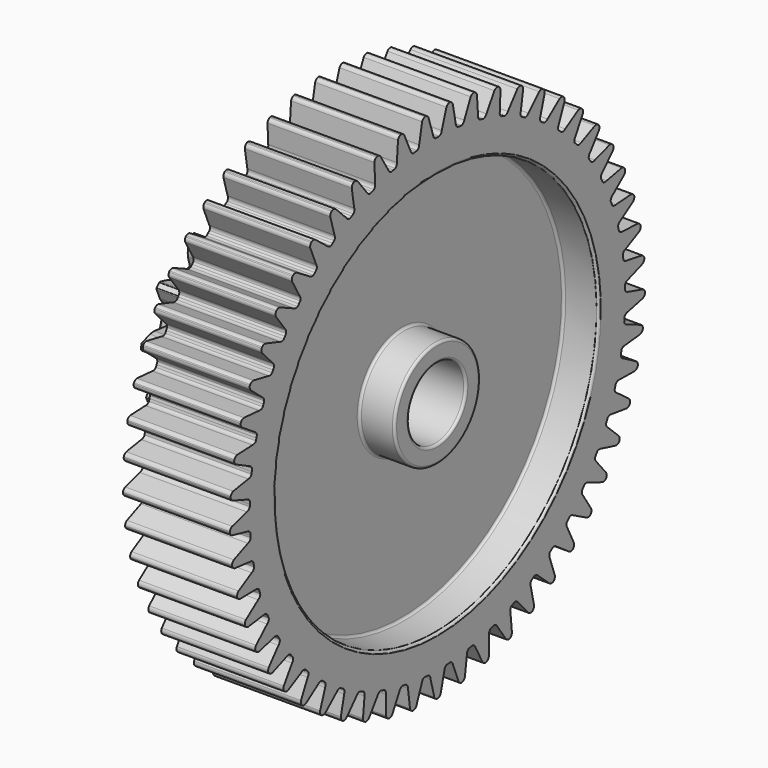
from build123d import *

# Parameters (mm, degrees)
F2_R            = 0.2
F4_DEPTH        = 13
F5_COUNT        = 11
F7_DEPTH        = 9
F7_COPIES_COUNT = 53


# Not quite as in the source:
# - a feature of the source that left no trace in its solid (it failed there, or was rolled back) is left out
# - a pattern or mirror of a feature is missing from the dataset's text; its kind, count and spacing are read off the source's solid


with BuildPart() as f1:
    # F0 (on Front) → F1 (revolve)
    with BuildSketch(Plane.XZ):
        Polygon((0, 17), (0, 21.85), (-9, 21.85), (-9, 17), (-6, 17), (-6, 7.5), (-19, 7.5), (-19, 4.4), (-20, 4.4), (-20, 3), (-19, 3), (0, 3), (0, 4.5), (-3, 4.5), (-3, 17), align=None)
    revolve(axis=Axis((-11.534338817, 0, 0), (-1, 0, 0)))

    # F2
    f2_edges = [f1.edges().sort_by_distance(p)[0] for p in [
        (0, 0, -3),
        (-19, 0, -4.4),
        (0, 0, -4.5),
        (-3, 0, -17),
        (0, 0, -17),
        (-6, 0, -17),
        (-9, 0, -17),
        (-20, 0, -4.4),
        (-20, 0, -3),
        (-3, 0, -4.5),
    ]]
    fillet(f2_edges, radius=F2_R)

    # F3 (on face) → F4 (cut)
    with BuildSketch(Plane(origin=(-19, 0, 0), x_dir=(0, -1, 0), z_dir=(-1, 0, 0))):
        with BuildLine():
            ThreePointArc((0.9908004602, 6.1770355537), (1.0982505044, 6.3805031544), (1.2301102445, 6.5690703453))
            Line((1.2301102445, 6.5690703453), (1.8030497794, 7.1902463429))
            ThreePointArc((1.8030497794, 7.1902463429), (1.8590461796, 7.2313431591), (1.9263826767, 7.2483825632))
            ThreePointArc((1.9263826767, 7.2483825632), (0, 7.5), (-1.9263826767, 7.2483825632))
            ThreePointArc((-1.9263826767, 7.2483825632), (-1.8590461796, 7.2313431591), (-1.8030497794, 7.1902463429))
            Line((-1.8030497794, 7.1902463429), (-1.2301102445, 6.5690703453))
            ThreePointArc((-1.2301102445, 6.5690703453), (-1.0982505044, 6.3805031544), (-0.9908004602, 6.1770355537))
            Line((-0.9908004602, 6.1770355537), (-0.6560313796, 5.1467222657))
            ThreePointArc((-0.6560313796, 5.1467222657), (-0.405230292, 4.8039981048), (0, 4.6769176328))
            ThreePointArc((0, 4.6769176328), (0.405230292, 4.8039981048), (0.6560313796, 5.1467222657))
            Line((0.6560313796, 5.1467222657), (0.9908004602, 6.1770355537))
        make_face()
    f4 = extrude(amount=-F4_DEPTH, mode=Mode.SUBTRACT)

    # F5: F4 ×11 about axis
    f5_axis = Axis((-6, 0, 0), (1, 0, 0))
    for i in range(1, F5_COUNT):
        add(f4.rotate(f5_axis, i * 360 / F5_COUNT), mode=Mode.SUBTRACT)

    # F6 (on face) → F7 (cut)
    with BuildSketch(Plane.YZ):
        with BuildLine():
            ThreePointArc((0, 19.75), (0.1013113163, 19.7497401506), (0.2026199667, 19.7489606093))
            ThreePointArc((0.2026199667, 19.7489606093), (0.3715580552, 19.8724239212), (0.4539108824, 20.0647810864))
            Line((0.4539108824, 20.0647810864), (0.9454404152, 21.5922750493))
            ThreePointArc((0.9454404152, 21.5922750493), (1.0699461505, 21.7413584659), (1.25, 21.8142155486))
            ThreePointArc((1.25, 21.8142155486), (0, 21.85), (-1.25, 21.8142155486))
            ThreePointArc((-1.25, 21.8142155486), (-1.0699461505, 21.7413584659), (-0.9454404152, 21.5922750493))
            Line((-0.9454404152, 21.5922750493), (-0.4539108824, 20.0647810864))
            ThreePointArc((-0.4539108824, 20.0647810864), (-0.3715580552, 19.8724239212), (-0.2026199667, 19.7489606093))
            ThreePointArc((-0.2026199667, 19.7489606093), (-0.1013113163, 19.7497401506), (0, 19.75))
        make_face()
    f7 = extrude(amount=-F7_DEPTH, mode=Mode.SUBTRACT)

    # F7_copies: F7 ×53 about axis
    f7_copies_axis = Axis((0, 0, 0), (1, 0, 0))
    for i in range(1, F7_COPIES_COUNT):
        add(f7.rotate(f7_copies_axis, i * 360 / F7_COPIES_COUNT), mode=Mode.SUBTRACT)


solid = f1.part
